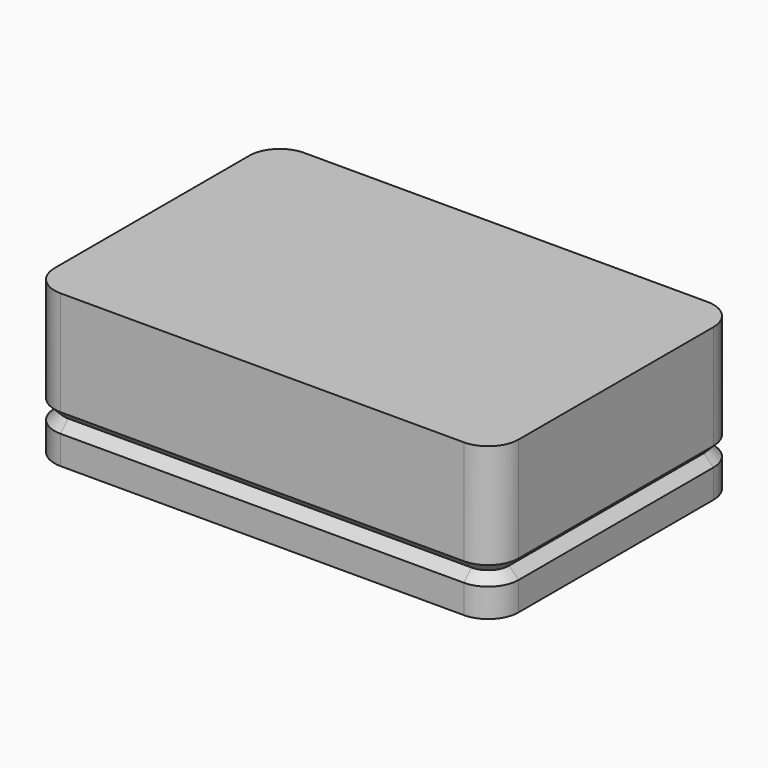
from build123d import *

# Parameters (mm, degrees)
F0_W       = 77.47
F0_H       = 50.8
F1_DEPTH   = 19.05
F2_W       = 58.42
F2_H       = 6.35
F2_H_2     = 19.05
F3_DEPTH   = 15.875
F2_R       = 1.5875
F2_W_2     = 6.35
F4_DEPTH   = 12.7
F2_W_3     = 3.175
F5_DEPTH   = 12.7
F6_SIZE    = 3.175
F7_W       = 77.47
F7_H       = 50.8
F7_W_2     = 64.77
F7_H_2     = 38.1
F8_DEPTH   = 19.05
F9_W       = 77.47
F9_H       = 50.8
F9_W_2     = 64.77
F9_H_2     = 38.1
F10_DEPTH  = 6.096
F11_R      = 5.08
F11_2_R    = 5.08
F12_DEPTH  = 15.875
F13_SIZE   = 1.58749
F13_2_SIZE = 1.58749
F14_R      = 1.5875
F15_DEPTH  = 3.175


# Not quite as in the source:
# - a fillet or chamfer is up to 0.001 mm smaller than in the source, because OpenCascade refuses the exact size


with BuildPart() as f1:
    # F0 (on Top) → F1 (new body)
    with BuildSketch(Plane.XY):
        Rectangle(F0_W, F0_H)
    extrude(amount=F1_DEPTH)

    # F2 (on face) → F3 (cut)
    with BuildSketch(Plane.XY.offset(19.05)):
        with Locations((0, -12.7)):
            Rectangle(F2_W, F2_H)
        Rectangle(F2_W, F2_H_2)
        with Locations((0, 12.7)):
            Rectangle(F2_W, F2_H)
    extrude(amount=-F3_DEPTH, mode=Mode.SUBTRACT)

    # F2 (on face) → F4 (cut)
    with BuildSketch(Plane.XY.offset(19.05)):
        Polygon((38.735, -9.525), (32.385, -9.525), (32.385, -19.05), (-32.385, -19.05), (-32.385, -9.525), (-38.735, -9.525), (-38.735, -25.4), (38.735, -25.4), align=None)
        with Locations((0, -22.225)):
            Circle(F2_R, mode=Mode.SUBTRACT)
        Polygon((32.385, 19.05), (32.385, 9.525), (38.735, 9.525), (38.735, 25.4), (-38.735, 25.4), (-38.735, 9.525), (-32.385, 9.525), (-32.385, 19.05), align=None)
        with Locations((0, 22.225)):
            Circle(F2_R, mode=Mode.SUBTRACT)
        with Locations((-35.56, 0)):
            Rectangle(F2_W_2, F2_H_2)
        with Locations((35.56, 0)):
            Rectangle(F2_W_2, F2_H_2)
        with Locations((0, 22.225)):
            Circle(F2_R)
        with Locations((0, -22.225)):
            Circle(F2_R)
    extrude(amount=-F4_DEPTH, mode=Mode.SUBTRACT)

    # F2 (on face) → F5 (cut)
    with BuildSketch(Plane.XY.offset(19.05)):
        with Locations((-35.56, 0)):
            Rectangle(F2_W_2, F2_H_2)
        with Locations((-30.7975, 0)):
            Rectangle(F2_W_3, F2_H_2)
        with Locations((30.7975, 0)):
            Rectangle(F2_W_3, F2_H_2)
        with Locations((35.56, 0)):
            Rectangle(F2_W_2, F2_H_2)
    extrude(amount=-F5_DEPTH, mode=Mode.SUBTRACT)

    # F6
    f6_edges = [f1.edges().sort_by_distance(p)[0] for p in [
        (-30.7975, 9.525, 19.05),
        (-30.7975, -9.525, 19.05),
        (30.7975, 9.525, 19.05),
        (30.7975, -9.525, 19.05),
    ]]
    chamfer(f6_edges, length=F6_SIZE)

    # F11
    f11_edges = [f1.edges().sort_by_distance(p)[0] for p in [
        (-38.735, 25.4, 3.175),
        (-38.735, -25.4, 3.175),
        (38.735, 25.4, 3.175),
        (38.735, -25.4, 3.175),
    ]]
    fillet(f11_edges, radius=F11_R)

    # F2 (on face) → F12 (cut)
    with BuildSketch(Plane.XY.offset(19.05)):
        with Locations((0, 22.225)):
            Circle(F2_R)
        with Locations((0, -22.225)):
            Circle(F2_R)
    extrude(amount=-F12_DEPTH, mode=Mode.SUBTRACT)

    # F13 (size 1.5875 in the source; OpenCascade refuses exactly that, so slightly less here)
    f13_edges = [f1.edges().sort_by_distance(p)[0] for p in [
        (0, 25.4, 6.35),
        (-38.735, 0, 6.35),
        (38.735, 0, 6.35),
        (37.247102, 23.912102, 6.35),
        (37.247102, -23.912102, 6.35),
        (0, -25.4, 6.35),
        (-37.247102, 23.912102, 6.35),
        (-37.247102, -23.912102, 6.35),
    ]]
    chamfer(f13_edges, length=F13_SIZE)


with BuildPart() as f8:
    # F7 (on face) → F8 (new body)
    with BuildSketch(Plane.XY.offset(6.35)):
        Rectangle(F7_W, F7_H)
        Rectangle(F7_W_2, F7_H_2, mode=Mode.SUBTRACT)
    extrude(amount=F8_DEPTH)

    # F9 (on face) → F10 (join)
    with BuildSketch(Plane.XY.offset(25.4)):
        Rectangle(F9_W, F9_H)
        Rectangle(F9_W_2, F9_H_2, mode=Mode.SUBTRACT)
        Rectangle(F9_W_2, F9_H_2)
    extrude(amount=-F10_DEPTH)

    # F11#2
    f11_2_edges = [f8.edges().sort_by_distance(p)[0] for p in [
        (-38.735, 25.4, 15.875),
        (-38.735, -25.4, 15.875),
        (38.735, 25.4, 15.875),
        (38.735, -25.4, 15.875),
    ]]
    fillet(f11_2_edges, radius=F11_2_R)

    # F13#2 (size 1.5875 in the source; OpenCascade refuses exactly that, so slightly less here)
    f13_2_edges = [f8.edges().sort_by_distance(p)[0] for p in [
        (0, 25.4, 6.35),
        (-38.735, 0, 6.35),
        (0, 19.05, 6.35),
        (-32.385, 0, 6.35),
        (0, -19.05, 6.35),
        (32.385, 0, 6.35),
        (38.735, 0, 6.35),
        (37.247102, 23.912102, 6.35),
        (37.247102, -23.912102, 6.35),
        (0, -25.4, 6.35),
        (-37.247102, 23.912102, 6.35),
        (-37.247102, -23.912102, 6.35),
    ]]
    chamfer(f13_2_edges, length=F13_2_SIZE)

    # F14 (on face) → F15 (cut)
    with BuildSketch(Plane.XY.offset(6.35)):
        with Locations((0, 22.225)):
            Circle(F14_R)
        with Locations((0, -22.225)):
            Circle(F14_R)
    extrude(amount=F15_DEPTH, mode=Mode.SUBTRACT)


solid = Compound([f1.part, f8.part])
